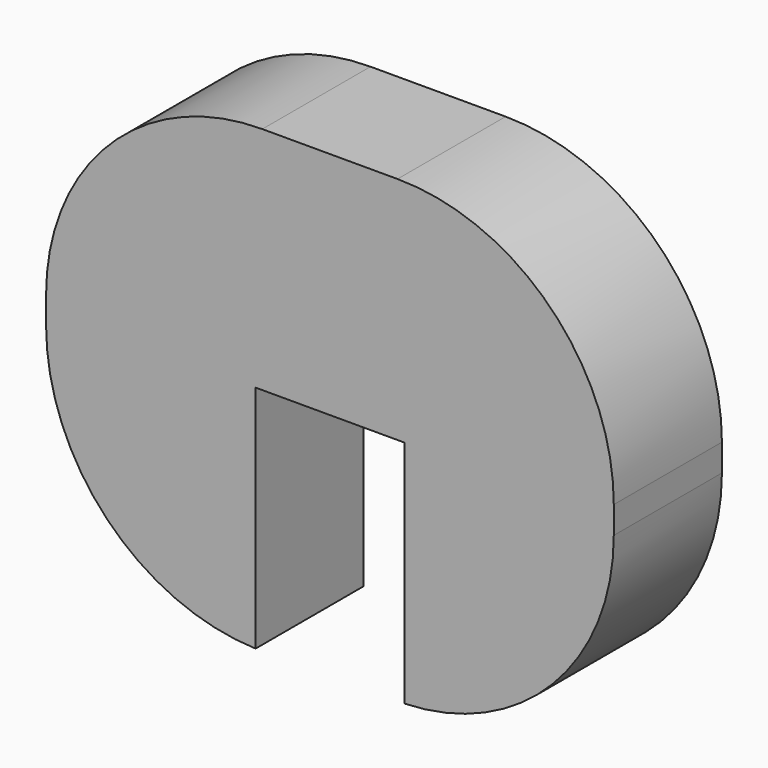
from build123d import *

# Parameters (mm, degrees)
F1_DEPTH    = 5
F2_T1_DEPTH = 45
F2_T3_DEPTH = 44.9804639793


# Not quite as in the source:
# - a fillet or chamfer that OpenCascade refuses, or shapes differently, is made with other operations: its cross-section is extruded or revolved along the edge and cut away or added


with BuildPart() as f1:
    # F0 (on Front) → F1 (new body)
    with BuildSketch(Plane.XZ):
        Polygon((2.75, -8.5), (10.5, -8.5), (10.5, 8.5), (-10.5, 8.5), (-10.5, -8.5), (-2.75, -8.5), (-2.75, 0), (2.75, 0), align=None)
    extrude(amount=F1_DEPTH)

    # F2: fillet of radius 8 on 4 edges, made by hand

    # F2_s2 → F2_t1 (cut)
    with BuildSketch(Plane.XZ.offset(-20)):
        with BuildLine():
            ThreePointArc((-2.5, 8.5), (-8.1568542495, 6.1568542495), (-10.5, 0.5))
            Line((-10.5, 0.5), (-10.5, 8.5))
            Line((-10.5, 8.5), (-2.5, 8.5))
        make_face()
        with BuildLine():
            ThreePointArc((10.5, 0.5), (8.1568542495, 6.1568542495), (2.5, 8.5))
            Line((2.5, 8.5), (10.5, 8.5))
            Line((10.5, 8.5), (10.5, 0.5))
        make_face()
    extrude(amount=F2_T1_DEPTH, mode=Mode.SUBTRACT)

    # F2_s4 → F2_t3 (cut)
    with BuildSketch(Plane.XZ.offset(-19.9902319896)):
        with BuildLine():
            ThreePointArc((2.75, -8.5), (8.2445626465, -6.071671567), (10.5, -0.5039072041))
            Line((10.5, -0.5039072041), (10.5, -8.5))
            Line((10.5, -8.5), (2.75, -8.5))
        make_face()
        with BuildLine():
            ThreePointArc((-10.5, -0.5039072041), (-8.2445626465, -6.071671567), (-2.75, -8.5))
            Line((-2.75, -8.5), (-10.5, -8.5))
            Line((-10.5, -8.5), (-10.5, -0.5039072041))
        make_face()
    extrude(amount=F2_T3_DEPTH, mode=Mode.SUBTRACT)


solid = f1.part
